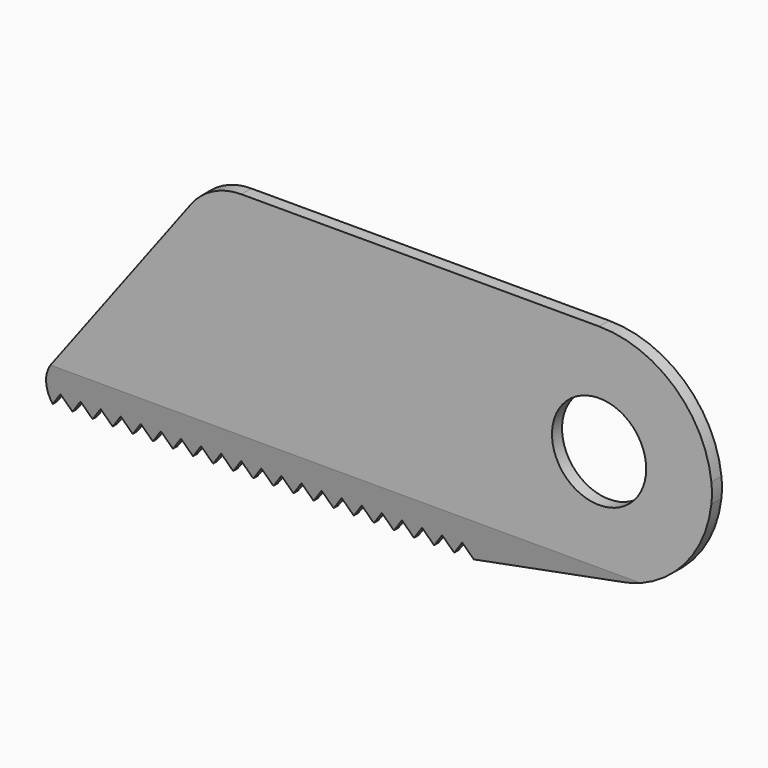
from build123d import *

# Parameters (mm, degrees)
F0_R           = 3.75
F1_DEPTH       = 1
F2_R           = 5
F3_R           = 1
F5_DEPTH       = 25
F7_DEPTH       = 25
F8_T1_DEPTH    = 10.2705098312
F10_DEPTH      = 30
F10_DEPTH_BACK = 25


# Not quite as in the source:
# - a fillet or chamfer that OpenCascade refuses, or shapes differently, is made with other operations: its cross-section is extruded or revolved along the edge and cut away or added


with BuildPart() as f1:
    # F0 (on Front) → F1 (new body)
    with BuildSketch(Plane.XZ):
        with BuildLine():
            Line((-27.5, -10), (7.9370479853, -10))
            Line((7.9370479853, -10), (20.3712052174, -7.3570382915))
            ThreePointArc((20.3712052174, -7.3570382915), (25.1669262461, -4.5995427), (27.4438066413, 0.4421373561))
            ThreePointArc((27.4438066413, 0.4421373561), (27.487512587, 1.2231450576), (27.4438066413, 2.004152759))
            ThreePointArc((27.4438066413, 2.004152759), (24.4984425132, 7.7095966656), (18.5, 10))
            Line((18.5, 10), (-12.5, 10))
            Line((-12.5, 10), (-27.5, -10))
        make_face()
        with Locations((18.5, 1.2231450576)):
            Circle(F0_R, mode=Mode.SUBTRACT)
    extrude(amount=F1_DEPTH)

    # F2
    f2_edges = [f1.edges().sort_by_distance(p)[0] for p in [
        (-12.5, -0.5, 10),
    ]]
    fillet(f2_edges, radius=F2_R)

    # F3
    f3_edges = [f1.edges().sort_by_distance(p)[0] for p in [
        (-27.5, -0.5, -10),
    ]]
    fillet(f3_edges, radius=F3_R)

    # F4 (on face) → F5 (cut)
    with BuildSketch(Plane.XZ.offset(1)):
        Polygon((-24.7211863589, -8.9615818119), (-25.5, -10), (-25.5, -14.0343736857), (7.9370479853, -14.0343736857), (8.0576272821, -10), (7.2788136411, -8.9615818119), (6.5, -10), (6.4576272821, -10), (5.6788136411, -8.9615818119), (4.9, -10), (4.8576272821, -10), (4.0788136411, -8.9615818119), (3.3, -10), (3.2576272821, -10), (2.4788136411, -8.9615818119), (1.7, -10), (1.6576272821, -10), (0.8788136411, -8.9615818119), (0.1, -10), (0.0576272821, -10), (-0.7211863589, -8.9615818119), (-1.5, -10), (-1.5423727179, -10), (-2.3211863589, -8.9615818119), (-3.1, -10), (-3.1423727179, -10), (-3.9211863589, -8.9615818119), (-4.7, -10), (-4.7423727179, -10), (-5.5211863589, -8.9615818119), (-6.3, -10), (-6.3423727179, -10), (-7.1211863589, -8.9615818119), (-7.9, -10), (-7.9423727179, -10), (-8.7211863589, -8.9615818119), (-9.5, -10), (-9.5423727179, -10), (-10.3211863589, -8.9615818119), (-11.1, -10), (-11.1423727179, -10), (-11.9211863589, -8.9615818119), (-12.7, -10), (-12.7423727179, -10), (-13.5211863589, -8.9615818119), (-14.3, -10), (-14.3423727179, -10), (-15.1211863589, -8.9615818119), (-15.9, -10), (-15.9423727179, -10), (-16.7211863589, -8.9615818119), (-17.5, -10), (-17.5423727179, -10), (-18.3211863589, -8.9615818119), (-19.1, -10), (-19.1423727179, -10), (-19.9211863589, -8.9615818119), (-20.7, -10), (-20.7423727179, -10), (-21.5211863589, -8.9615818119), (-22.3, -10), (-22.3423727179, -10), (-23.1211863589, -8.9615818119), (-23.9, -10), (-23.9423727179, -10), align=None)
    extrude(amount=-F5_DEPTH, mode=Mode.SUBTRACT)

    # F6 (on face) → F7 (cut)
    with BuildSketch(Plane.XZ.offset(1)):
        Polygon((-26.6561899334, -14.2840119079), (-25.5, -10), (-26.3, -8.4), (-30.4410159588, -7.8742252663), align=None)
    extrude(amount=-F7_DEPTH, mode=Mode.SUBTRACT)

    # F8: fillet of radius 3 on 1 edges, made by hand

    # F8_s2 → F8_t1 (cut)
    with BuildSketch(Plane.XZ.offset(-4.6352549156)):
        with BuildLine():
            ThreePointArc((-25.1875388203, -6.916718427), (-25.7754167621, -8.4473016411), (-25.4708203932, -10.0583592135))
            Line((-25.4708203932, -10.0583592135), (-26.3, -8.4))
            Line((-26.3, -8.4), (-25.1875388203, -6.916718427))
        make_face()
    extrude(amount=F8_T1_DEPTH, mode=Mode.SUBTRACT)

    # F9 (on Right) → F10 (cut, two sides)
    with BuildSketch(Plane.YZ) as f10_sk:
        Polygon((-2.5567745324, -10.8186043799), (-0.4, -10), (-1, -6.9173601342), (-2.5567745324, -6.9173601342), align=None)
    extrude(amount=-F10_DEPTH, mode=Mode.SUBTRACT)
    extrude(f10_sk.sketch, amount=F10_DEPTH_BACK, mode=Mode.SUBTRACT)


solid = f1.part
